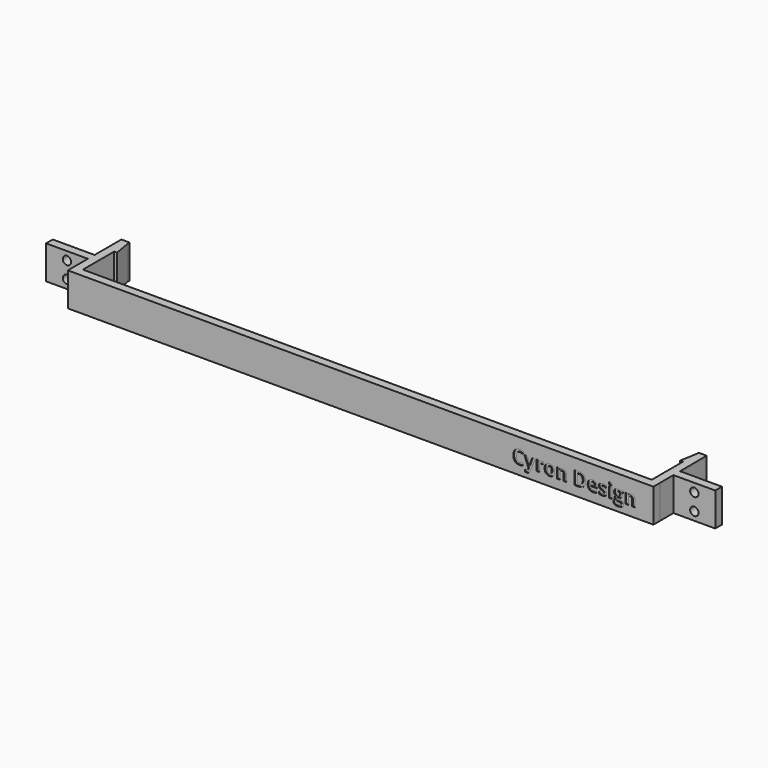
from build123d import *

# Parameters (mm, degrees)
F1_START     = 1
F0_W         = 5
F0_H         = 1
F1_DEPTH     = 4
F3_D         = 1
F5_D         = 1
F6_TEXT_SIZE = 2.2648613796
F7_DEPTH     = 0.1


# Not quite as in the source:
# - a feature names something its author has since deleted; it is built from what else it names
# - Text() gives the source's letters only with a copy of the font that has no kerning and outlines rounded to 1/6400 em; it was checked with that copy


with BuildPart() as f1:
    # F0 (on Top) → F1 (new body)
    with BuildSketch(Plane.XY.offset(F1_START)):
        with Locations((-37.5, -16.5119731403)):
            Rectangle(F0_W, F0_H)
        Polygon((-34, -12.3352976367), (-34, -12.0119731403), (-35, -12.0119731403), (-35, -16.0119731403), (-35, -17.0119731403), (-35, -19.0119731403), (-34, -19.0119731403), (-34, -14.3352976367), (-34, -12.401483839), align=None)
        Polygon((-34, -19.0119731403), (-35, -19.0119731403), (-35, -20.0119731403), (35, -20.0119731403), (35, -19.0119731403), (34, -19.0119731403), align=None)
        Polygon((34.9877508274, -16.0119981474), (34.9918338849, -17.0119898117), (39.9918330086, -17.0090295321), (39.9877499511, -16.0090378678), align=None)
        Polygon((34, -14.3352976367), (34, -19.0119731403), (35, -19.0119731403), (34.9918338849, -17.0119898117), (34.9877508274, -16.0119981474), (34.9714184612, -12.0119981474), (34, -12.0119731403), (34, -12.3352976367), align=None)
        Polygon((33.65, -14.3352976367), (34, -14.3352976367), (34, -12.3352976367), align=None)
        Polygon((-33.65, -14.3352976367), (-34, -12.3352976367), (-34, -12.401483839), (-34, -14.3352976367), align=None)
    extrude(amount=F1_DEPTH)

    # F3 (through all)
    with Locations(Plane.XZ.offset(17.0119731403)):
        with Locations((-37.5, 4), (-37.5, 2)):
            Hole(F3_D / 2)

    # F5 (through all)
    with Locations(Plane(origin=(0.0100843134, -17.0327009677, 0), x_dir=(0.9999998247, 0.0005920559, 0), z_dir=(0.0005920559, -0.9999998247, 0))):
        with Locations((37.4817557026, 2), (37.4817557026, 4)):
            Hole(F5_D / 2)

    # F6 (on face) → F7 (cut)
    with BuildSketch(Plane.XZ.offset(20.0119731403)):
        with Locations((18.1294246577, 2.0967689343)):
            Text('Cyron Design', F6_TEXT_SIZE, font='Open Sans', font_style=FontStyle.BOLD, text_align=(TextAlign.LEFT, TextAlign.BOTTOM))
    extrude(amount=-F7_DEPTH, mode=Mode.SUBTRACT)


solid = f1.part
